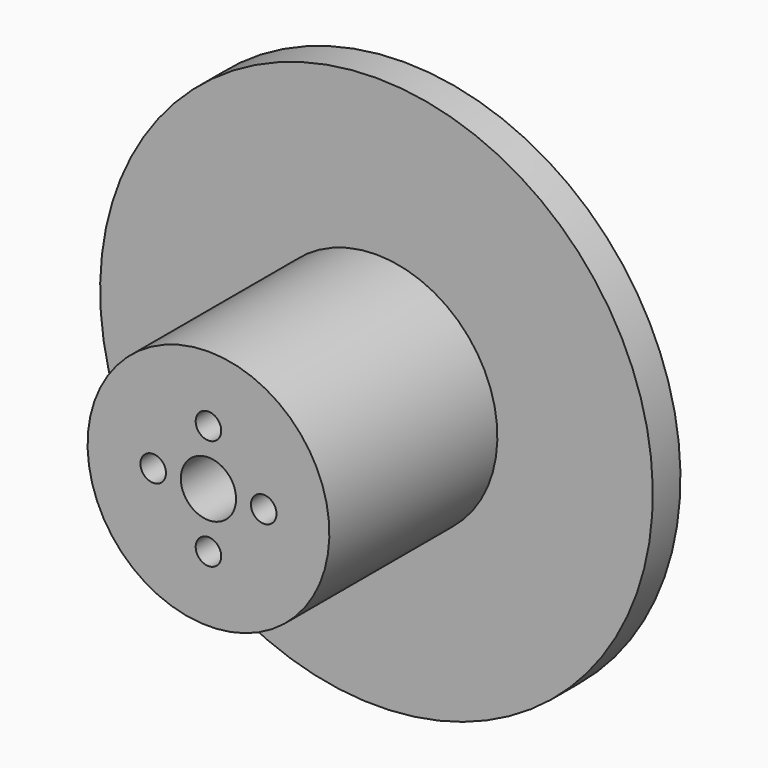
from build123d import *

# Parameters (mm, degrees)
F0_W     = 25.4
F0_H     = 17.5
F2_R     = 1.85
F2_R_2   = 4
F3_DEPTH = 40
F4_DEPTH = 5


# Not quite as in the source:
# - a feature names something its author has since deleted; it is built from what else it names


with BuildPart() as f1:
    # F0 (on Right) → F1 (revolve)
    with BuildSketch(Plane.YZ):
        with Locations((12.7, 8.75)):
            Rectangle(F0_W, F0_H)
        Polygon((25.4, 17.5), (25.4, 0), (30.4, 0), (30.4, 40), (25.4, 40), align=None)
    revolve(axis=Axis((0, 12.7, 0), (0, 1, 0)))

    # F2 (on face) → F3 (cut)
    with BuildSketch(Plane(origin=(0, 30.4, 0), x_dir=(-1, 0, 0), z_dir=(0, 1, 0))):
        with Locations((0, 8)):
            Circle(F2_R)
        with Locations((-8, 0)):
            Circle(F2_R)
        Circle(F2_R_2)
        with Locations((0, -8)):
            Circle(F2_R)
        with Locations((8, 0)):
            Circle(F2_R)
    extrude(amount=-F3_DEPTH, mode=Mode.SUBTRACT)

    # F4 (add): a face of the model
    f4_faces = [f1.faces().sort_by_distance(p)[0] for p in [
        (0, 0, -17.0050252532),
    ]]
    extrude(f4_faces, amount=F4_DEPTH)


solid = f1.part
